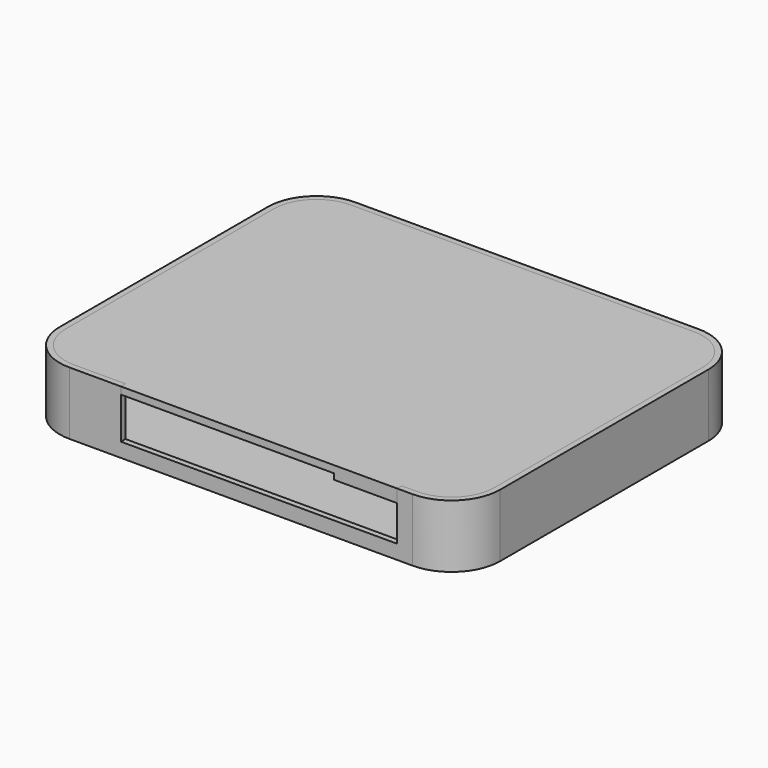
from build123d import *

# Parameters (mm, degrees)
F0_W      = 120
F0_H      = 110
F0_R      = 3.5
F0_R_2    = 1.5
F1_DEPTH  = 2
F2_DEPTH  = 20
F3_DEPTH  = 3
F4_DEPTH  = 10
F5_W      = 96.6
F5_H      = 2
F6_DEPTH  = 17
F7_R      = 1.5
F8_DEPTH  = 2
F9_W      = 1.8643289804
F9_H      = 63.8286471367
F9_W_2    = 2.3556724191
F9_H_2    = 58.8918318972
F10_DEPTH = 1
F9_W_3    = 74.5
F9_H_3    = 2
F11_DEPTH = 2.5
F9_W_4    = 22.1
F12_DEPTH = 4.5
F13_DEPTH = 20


with BuildPart() as f1:
    # F0 (on Top) → F1 (new body)
    with BuildSketch(Plane.XY):
        with BuildLine():
            Line((-77, 51), (-77, -40))
            ThreePointArc((-77, -40), (-72.0208152802, -52.0208152802), (-60, -57))
            Line((-60, -57), (60, -57))
            ThreePointArc((60, -57), (72.0208152802, -52.0208152802), (77, -40))
            Line((77, -40), (77, 51))
            ThreePointArc((77, 51), (72.0208152802, 63.0208152802), (60, 68))
            Line((60, 68), (-60, 68))
            ThreePointArc((-60, 68), (-72.0208152802, 63.0208152802), (-77, 51))
        make_face()
        with BuildLine():
            Line((60, -55), (-60, -55))
            ThreePointArc((-60, -55), (-70.6066017178, -50.6066017178), (-75, -40))
            Line((-75, -40), (-75, 51))
            ThreePointArc((-75, 51), (-70.6066017178, 61.6066017178), (-60, 66))
            Line((-60, 66), (60, 66))
            ThreePointArc((60, 66), (70.6066017178, 61.6066017178), (75, 51))
            Line((75, 51), (75, -40))
            ThreePointArc((75, -40), (70.6066017178, -50.6066017178), (60, -55))
        make_face(mode=Mode.SUBTRACT)
        Rectangle(F0_W, F0_H)
        with Locations((-55.5, -46)):
            Circle(F0_R, mode=Mode.SUBTRACT)
        with Locations((56, -39.5)):
            Circle(F0_R, mode=Mode.SUBTRACT)
        with Locations((-50, 45)):
            Circle(F0_R, mode=Mode.SUBTRACT)
        with Locations((56, 41)):
            Circle(F0_R, mode=Mode.SUBTRACT)
        with BuildLine():
            ThreePointArc((-75, -40), (-70.6066017178, -50.6066017178), (-60, -55))
            Line((-60, -55), (-60, 55))
            Line((-60, 55), (60, 55))
            Line((60, 55), (60, -55))
            ThreePointArc((60, -55), (70.6066017178, -50.6066017178), (75, -40))
            Line((75, -40), (75, 51))
            ThreePointArc((75, 51), (70.6066017178, 61.6066017178), (60, 66))
            Line((60, 66), (-60, 66))
            ThreePointArc((-60, 66), (-70.6066017178, 61.6066017178), (-75, 51))
            Line((-75, 51), (-75, -40))
        make_face()
        Polygon((-68.426687021, -2.8152682781), (-66.426687021, -2.8152682781), (-66.426687021, 1.1847317219), (-64.77445364, 1.1847317219), (-64.77445364, -6.8152682781), (-70.078920402, -6.8152682781), (-70.078920402, 1.1847317219), (-68.426687021, 1.1847317219), align=None, mode=Mode.SUBTRACT)
        Polygon((-68.426687021, 45.6847317219), (-70.078920402, 45.6847317219), (-70.078920402, 53.6847317219), (-64.77445364, 53.6847317219), (-64.77445364, 45.6847317219), (-66.426687021, 45.6847317219), (-66.426687021, 49.6847317219), (-68.426687021, 49.6847317219), align=None, mode=Mode.SUBTRACT)
        Polygon((11.0850978998, 61.4750083983), (6.792485714, 61.4750083983), (6.792485714, 59.4750083983), (11.0850978998, 59.4750083983), (11.0850978998, 57.4750083983), (3.0850978998, 57.4750083983), (3.0850978998, 63.4750083983), (11.0850978998, 63.4750083983), align=None, mode=Mode.SUBTRACT)
        Polygon((59.292485714, 59.4750083983), (59.292485714, 61.4750083983), (54.4998735282, 61.4750083983), (54.4998735282, 63.4750083983), (62.4998735282, 63.4750083983), (62.4998735282, 57.4750083983), (54.9998735282, 57.4750083983), (54.9998735282, 59.4750083983), align=None, mode=Mode.SUBTRACT)
        Polygon((6.792485714, 59.4750083983), (6.792485714, 61.4750083983), (11.0850978998, 61.4750083983), (11.0850978998, 63.4750083983), (3.0850978998, 63.4750083983), (3.0850978998, 57.4750083983), (11.0850978998, 57.4750083983), (11.0850978998, 59.4750083983), align=None)
        with Locations((56, -39.5)):
            Circle(F0_R)
        with Locations((56, -39.5)):
            Circle(F0_R_2, mode=Mode.SUBTRACT)
        with Locations((-50, 45)):
            Circle(F0_R)
        with Locations((-50, 45)):
            Circle(F0_R_2, mode=Mode.SUBTRACT)
        with Locations((56, 41)):
            Circle(F0_R)
        with Locations((56, 41)):
            Circle(F0_R_2, mode=Mode.SUBTRACT)
        with Locations((-55.5, -46)):
            Circle(F0_R)
        with Locations((-55.5, -46)):
            Circle(F0_R_2, mode=Mode.SUBTRACT)
        Polygon((54.4998735282, 61.4750083983), (59.292485714, 61.4750083983), (59.292485714, 59.4750083983), (54.9998735282, 59.4750083983), (54.9998735282, 57.4750083983), (62.4998735282, 57.4750083983), (62.4998735282, 63.4750083983), (54.4998735282, 63.4750083983), align=None)
        Polygon((-70.078920402, 53.6847317219), (-70.078920402, 45.6847317219), (-68.426687021, 45.6847317219), (-68.426687021, 49.6847317219), (-66.426687021, 49.6847317219), (-66.426687021, 45.6847317219), (-64.77445364, 45.6847317219), (-64.77445364, 53.6847317219), align=None)
        Polygon((-66.426687021, 1.1847317219), (-66.426687021, -2.8152682781), (-68.426687021, -2.8152682781), (-68.426687021, 1.1847317219), (-70.078920402, 1.1847317219), (-70.078920402, -6.8152682781), (-64.77445364, -6.8152682781), (-64.77445364, 1.1847317219), align=None)
        with Locations((-55.5, -46)):
            Circle(F0_R_2)
        with Locations((56, 41)):
            Circle(F0_R_2)
        with Locations((-50, 45)):
            Circle(F0_R_2)
        with Locations((56, -39.5)):
            Circle(F0_R_2)
    extrude(amount=-F1_DEPTH)

    # F0 (on Top) → F2 (join)
    with BuildSketch(Plane.XY):
        with BuildLine():
            Line((-77, 51), (-77, -40))
            ThreePointArc((-77, -40), (-72.0208152802, -52.0208152802), (-60, -57))
            Line((-60, -57), (60, -57))
            ThreePointArc((60, -57), (72.0208152802, -52.0208152802), (77, -40))
            Line((77, -40), (77, 51))
            ThreePointArc((77, 51), (72.0208152802, 63.0208152802), (60, 68))
            Line((60, 68), (-60, 68))
            ThreePointArc((-60, 68), (-72.0208152802, 63.0208152802), (-77, 51))
        make_face()
        with BuildLine():
            Line((60, -55), (-60, -55))
            ThreePointArc((-60, -55), (-70.6066017178, -50.6066017178), (-75, -40))
            Line((-75, -40), (-75, 51))
            ThreePointArc((-75, 51), (-70.6066017178, 61.6066017178), (-60, 66))
            Line((-60, 66), (60, 66))
            ThreePointArc((60, 66), (70.6066017178, 61.6066017178), (75, 51))
            Line((75, 51), (75, -40))
            ThreePointArc((75, -40), (70.6066017178, -50.6066017178), (60, -55))
        make_face(mode=Mode.SUBTRACT)
    extrude(amount=F2_DEPTH)

    # F0 (on Top) → F3 (join)
    with BuildSketch(Plane.XY):
        with Locations((-50, 45)):
            Circle(F0_R)
        with Locations((-50, 45)):
            Circle(F0_R_2, mode=Mode.SUBTRACT)
        with Locations((56, 41)):
            Circle(F0_R)
        with Locations((56, 41)):
            Circle(F0_R_2, mode=Mode.SUBTRACT)
        with Locations((56, -39.5)):
            Circle(F0_R)
        with Locations((56, -39.5)):
            Circle(F0_R_2, mode=Mode.SUBTRACT)
        with Locations((-55.5, -46)):
            Circle(F0_R)
        with Locations((-55.5, -46)):
            Circle(F0_R_2, mode=Mode.SUBTRACT)
    extrude(amount=F3_DEPTH)

    # F0 (on Top) → F4 (join)
    with BuildSketch(Plane.XY):
        Polygon((6.792485714, 59.4750083983), (6.792485714, 61.4750083983), (11.0850978998, 61.4750083983), (11.0850978998, 63.4750083983), (3.0850978998, 63.4750083983), (3.0850978998, 57.4750083983), (11.0850978998, 57.4750083983), (11.0850978998, 59.4750083983), align=None)
        Polygon((54.4998735282, 61.4750083983), (59.292485714, 61.4750083983), (59.292485714, 59.4750083983), (54.9998735282, 59.4750083983), (54.9998735282, 57.4750083983), (62.4998735282, 57.4750083983), (62.4998735282, 63.4750083983), (54.4998735282, 63.4750083983), align=None)
        Polygon((-66.426687021, 1.1847317219), (-66.426687021, -2.8152682781), (-68.426687021, -2.8152682781), (-68.426687021, 1.1847317219), (-70.078920402, 1.1847317219), (-70.078920402, -6.8152682781), (-64.77445364, -6.8152682781), (-64.77445364, 1.1847317219), align=None)
        Polygon((-70.078920402, 53.6847317219), (-70.078920402, 45.6847317219), (-68.426687021, 45.6847317219), (-68.426687021, 49.6847317219), (-66.426687021, 49.6847317219), (-66.426687021, 45.6847317219), (-64.77445364, 45.6847317219), (-64.77445364, 53.6847317219), align=None)
    extrude(amount=F4_DEPTH)

    # F5 (on face) → F6 (cut, through all)
    with BuildSketch(Plane.XY.offset(20)):
        with Locations((6.3, -56)):
            Rectangle(F5_W, F5_H)
    extrude(amount=-F6_DEPTH, mode=Mode.SUBTRACT)

    # F7 (on face) → F8 (cut, through all)
    with BuildSketch(Plane(origin=(0, 68, 0), x_dir=(-1, 0, 0), z_dir=(0, 1, 0))):
        with Locations((2.5, 8)):
            Circle(F7_R)
        with Locations((13.5, 8)):
            Circle(F7_R)
        with Locations((24.5, 8)):
            Circle(F7_R)
        with Locations((44.5, 8)):
            Circle(F7_R)
    extrude(amount=-F8_DEPTH, mode=Mode.SUBTRACT)


with BuildPart() as f10:
    # F9 (on face) → F10 (new body)
    with BuildSketch(Plane.XY.offset(20)):
        with BuildLine():
            Line((-75, 51), (-75, -40))
            ThreePointArc((-75, -40), (-70.6066017178, -50.6066017178), (-60, -55))
            Line((-60, -55), (-42, -55))
            Line((-42, -55), (32.5, -55))
            Line((32.5, -55), (54.6, -55))
            Line((54.6, -55), (60, -55))
            ThreePointArc((60, -55), (70.6066017178, -50.6066017178), (75, -40))
            Line((75, -40), (75, 51))
            ThreePointArc((75, 51), (70.6066017178, 61.6066017178), (60, 66))
            Line((60, 66), (-60, 66))
            ThreePointArc((-60, 66), (-70.6066017178, 61.6066017178), (-75, 51))
        make_face()
        with Locations((-72.3674446344, 16.4873562753)):
            Rectangle(F9_W, F9_H, mode=Mode.SUBTRACT)
        with Locations((67.2655664384, 20.6032958813)):
            Rectangle(F9_W_2, F9_H_2, mode=Mode.SUBTRACT)
    extrude(amount=-F10_DEPTH)

    # F9 (on face) → F11 (join)
    with BuildSketch(Plane.XY.offset(20)):
        with Locations((-4.75, -56)):
            Rectangle(F9_W_3, F9_H_3)
    extrude(amount=-F11_DEPTH)

    # F9 (on face) → F12 (join)
    with BuildSketch(Plane.XY.offset(20)):
        with Locations((43.55, -56)):
            Rectangle(F9_W_4, F9_H_3)
    extrude(amount=-F12_DEPTH)

    # F9 (on face) → F13 (join, through all)
    with BuildSketch(Plane.XY.offset(20)):
        with Locations((-72.3674446344, 16.4873562753)):
            Rectangle(F9_W, F9_H)
        with Locations((67.2655664384, 20.6032958813)):
            Rectangle(F9_W_2, F9_H_2)
    extrude(amount=-F13_DEPTH)


solid = Compound([f1.part, f10.part])
